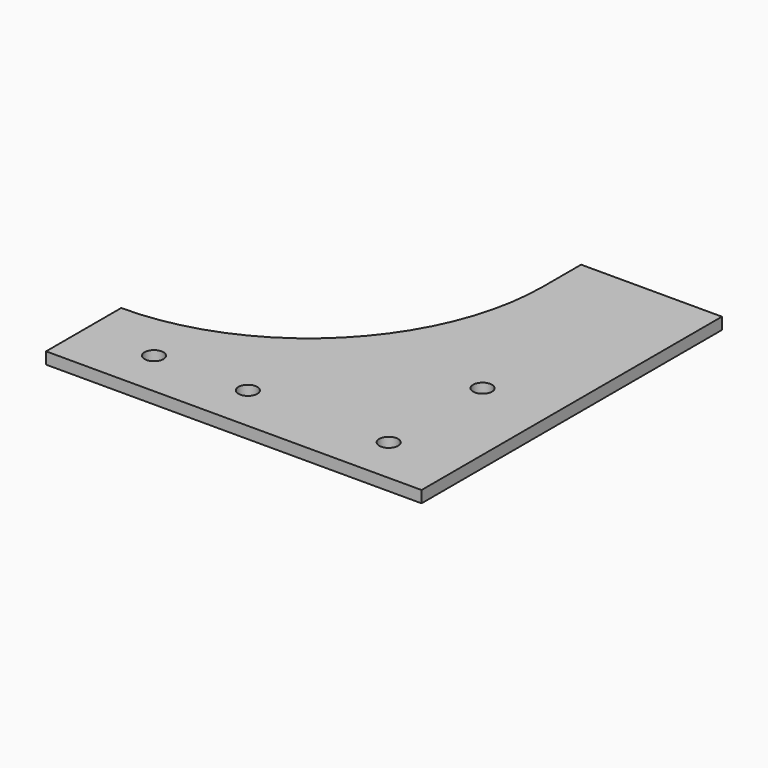
from build123d import *

# Parameters (mm, degrees)
F1_DEPTH = 3.175
F2_R     = 63.49999
F3_D     = 5.1054


# Not quite as in the source:
# - a fillet or chamfer is up to 0.001 mm smaller than in the source, because OpenCascade refuses the exact size


with BuildPart() as f1:
    # F0 (on Top) → F1 (new body)
    with BuildSketch(Plane.XY):
        Polygon((-101.6, 0), (0, 0), (0, 101.6), (-38.1, 101.6), (-38.1, 25.4), (-101.6, 25.4), align=None)
    extrude(amount=F1_DEPTH)

    # F2 (radius 63.5 in the source; OpenCascade refuses exactly that, so slightly less here)
    f2_edges = [f1.edges().sort_by_distance(p)[0] for p in [
        (-38.1, 25.4, 1.5875),
    ]]
    fillet(f2_edges, radius=F2_R)

    # F3 (through all)
    with Locations(Plane(origin=(0, 0, 0), x_dir=(1, 0, 0), z_dir=(0, 0, -1))):
        with Locations((-82.55, -12.7), (-57.15, -12.7), (-19.05, -12.7), (-19.05, -44.45)):
            Hole(F3_D / 2)


solid = f1.part
